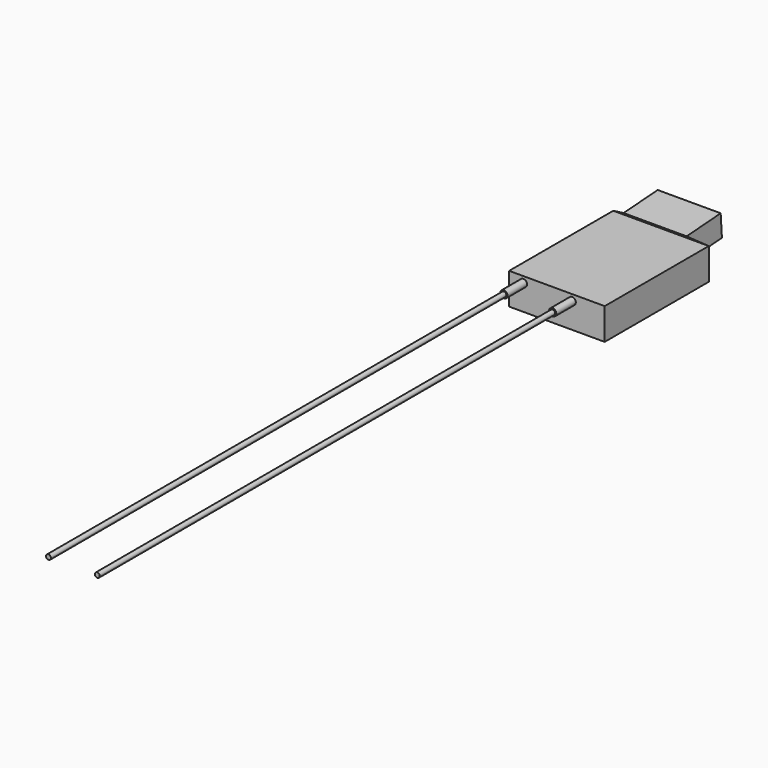
from build123d import *

# Parameters (mm, degrees)
F0_W      = 23.5
F0_H      = 32
F1_DEPTH  = 7.75
F4_W      = 15.5
F4_H      = 5.5
F5_DEPTH  = 10.5
F1_FACE_W = 23.5
F1_FACE_H = 7.75
F5_FACE_W = 15.5
F5_FACE_H = 5.5
F7_R      = 0.9
F8_DEPTH  = 6
F9_R      = 0.6
F10_DEPTH = 140


with BuildPart() as f1:
    # F0 (on Top) → F1 (new body)
    with BuildSketch(Plane.XY):
        Rectangle(F0_W, F0_H)
    extrude(amount=F1_DEPTH)



with BuildPart() as f5:
    # F4 (on face) → F5 (new body)
    with BuildSketch(Plane(origin=(0, 16.6609531262, 1.1650473361), x_dir=(-1, 0, 0), z_dir=(0, 0.9975640503, 0.0697564737))):
        with Locations((1.6, 4.0650178096)):
            Rectangle(F4_W, F4_H)
    extrude(amount=F5_DEPTH)


with BuildPart() as f1_1:
    add(f1.part)

    add(f5.part)  # F6 merges F5
    # F1_face (on face) → F6 section 0
    with BuildSketch(Plane(origin=(0, 16, 3.875), x_dir=(-1, 0, 0), z_dir=(0, 1, 0))):
        Rectangle(F1_FACE_W, F1_FACE_H)
    # F5_face (on face) → F6 section 1
    with BuildSketch(Plane(origin=(-1.6, 16.3773918181, 5.2201629666), x_dir=(-1, 0, 0), z_dir=(0, -0.9975640503, -0.0697564737))):
        Rectangle(F5_FACE_W, F5_FACE_H)
    loft()

    # F7 (on face) → F8 (join)
    with BuildSketch(Plane.XZ.offset(16)):
        with Locations((-8.25, 6.25)):
            Circle(F7_R)
        with Locations((3.75, 6.25)):
            Circle(F7_R)
    extrude(amount=F8_DEPTH)

    # F9 (on face) → F10 (join)
    with BuildSketch(Plane.XZ.offset(22)):
        with Locations((-8.25, 6.25)):
            Circle(F9_R)
        with Locations((3.75, 6.25)):
            Circle(F9_R)
    extrude(amount=F10_DEPTH)


solid = f1_1.part
